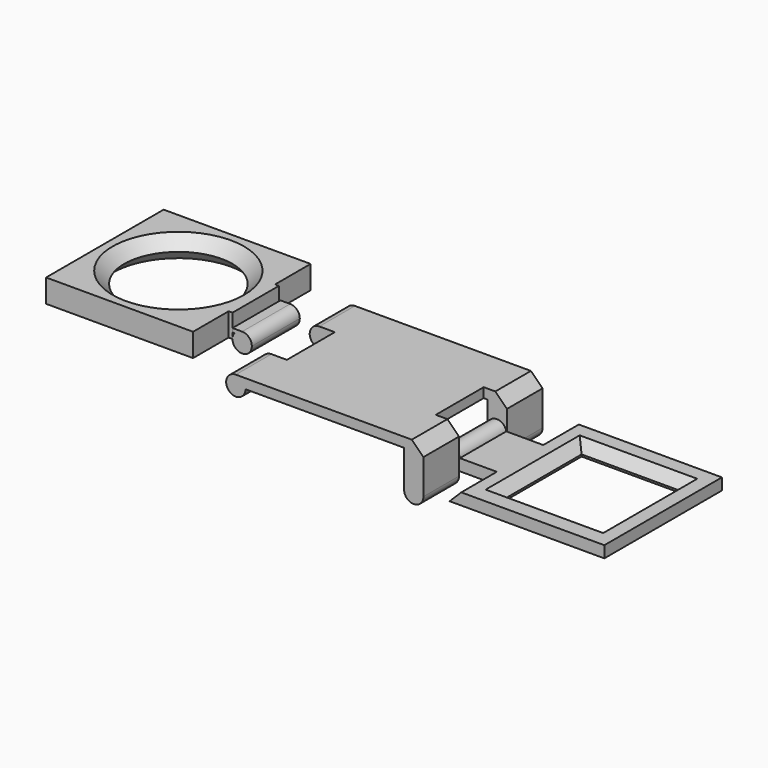
from build123d import *

# Parameters (mm, degrees)
F0_W      = 25.4
F0_H      = 25.4
F0_W_2    = 9
F0_H_2    = 15
F1_DEPTH  = 3
F2_SIZE   = 2.99999
F3_SIZE   = 2.5
F4_R      = 2.5
F5_DEPTH  = 15
F6_W      = 5
F6_H      = 11.5
F7_DEPTH  = 2.5
F8_DEPTH  = 12
F9_R      = 2.5
F10_DEPTH = 11.5
F11_R     = 2.5
F12_DEPTH = 11.5
F13_SIZE  = 3
F14_R     = 2.5
F15_DEPTH = 11.5
F16_R     = 2.5
F17_DEPTH = 11.5
F19_R     = 14
F19_W     = 1
F19_H     = 15
F20_DEPTH = 6
F22_DEPTH = 15.5
F23_SIZE  = 2.99999


# Not quite as in the source:
# - a fillet or chamfer is up to 0.001 mm smaller than in the source, because OpenCascade refuses the exact size


with BuildPart() as f1:
    # F0 (on Top) → F1 (new body)
    with BuildSketch(Plane.XY):
        Polygon((20, -19), (20, 19), (-20, 19), (-20, 7.5), (-20, -7.5), (-20, -19), align=None)
        with Locations((1.3, 0.2)):
            Rectangle(F0_W, F0_H, mode=Mode.SUBTRACT)
        with Locations((-24.5, 0)):
            Rectangle(F0_W_2, F0_H_2)
    extrude(amount=F1_DEPTH)

    # F2 (size 3 in the source; OpenCascade refuses exactly that, so slightly less here)
    f2_edges = [f1.edges().sort_by_distance(p)[0] for p in [
        (-20, -13.25, 3),
        (-20, 13.25, 3),
    ]]
    chamfer(f2_edges, length=F2_SIZE)

    # F3
    f3_edges = [f1.edges().sort_by_distance(p)[0] for p in [
        (1.3, 12.9, 3),
        (14, 0.2, 3),
        (1.3, -12.5, 3),
        (-11.4, 0.2, 3),
    ]]
    chamfer(f3_edges, length=F3_SIZE)

    # F4 (on face) → F5 (join)
    with BuildSketch(Plane.XZ.offset(7.5)):
        with Locations((-29, 2.5)):
            Circle(F4_R)
    extrude(amount=-F5_DEPTH)


with BuildPart() as f7:
    # F6 (on Top) → F7 (new body)
    with BuildSketch(Plane.XY):
        Polygon((19.25, 19.25), (-24.25, 19.25), (-24.25, 7.75), (-20.25, 7.75), (-20.25, -7.75), (-24.25, -7.75), (-24.25, -19.25), (19.25, -19.25), (19.25, -7.75), (18.25, -7.75), (18.25, 7.75), (19.25, 7.75), align=None)
        with Locations((21.75, -13.5)):
            Rectangle(F6_W, F6_H)
        with Locations((21.75, 13.5)):
            Rectangle(F6_W, F6_H)
    extrude(amount=-F7_DEPTH)

    # F6 (on Top) → F8 (join)
    with BuildSketch(Plane.XY):
        with Locations((21.75, -13.5)):
            Rectangle(F6_W, F6_H)
        with Locations((21.75, 13.5)):
            Rectangle(F6_W, F6_H)
    extrude(amount=-F8_DEPTH)

    # F9 (on face) → F10 (join)
    with BuildSketch(Plane.XZ.offset(19.25)):
        with Locations((21.75, -12)):
            Circle(F9_R)
    extrude(amount=-F10_DEPTH)

    # F11 (on face) → F12 (join)
    with BuildSketch(Plane(origin=(0, 19.25, 0), x_dir=(-1, 0, 0), z_dir=(0, 1, 0))):
        with Locations((-21.75, -12)):
            Circle(F11_R)
    extrude(amount=-F12_DEPTH)

    # F13
    f13_edges = [f7.edges().sort_by_distance(p)[0] for p in [
        (24.25, -13.5, 0),
        (24.25, 13.5, 0),
    ]]
    chamfer(f13_edges, length=F13_SIZE)

    # F14 (on face) → F15 (join)
    with BuildSketch(Plane.XZ.offset(19.25)):
        with Locations((-24.25, -2.5)):
            Circle(F14_R)
    extrude(amount=-F15_DEPTH)

    # F16 (on face) → F17 (join)
    with BuildSketch(Plane(origin=(0, 19.25, 0), x_dir=(-1, 0, 0), z_dir=(0, 1, 0))):
        with Locations((24.25, -2.5)):
            Circle(F16_R)
    extrude(amount=-F17_DEPTH)


with BuildPart() as f1_1:
    # F18: moved
    add(f1.part.moved(Location((50.83962, 0, -11))))


with BuildPart() as f20:
    # F19 (on Top) → F20 (new body)
    with BuildSketch(Plane.XY):
        Polygon((-35.5119029816, 7.5), (-35.5119029816, 19), (-73.5119029816, 19), (-73.5119029816, -19), (-35.5119029816, -19), (-35.5119029816, -7.5), (-36.5119029816, -7.5), (-36.5119029816, 7.5), align=None)
        with Locations((-54.5119029816, 0)):
            Circle(F19_R, mode=Mode.SUBTRACT)
        with Locations((-35.0119029816, 0)):
            Rectangle(F19_W, F19_H)
        with Locations((-36.0119029816, 0)):
            Rectangle(F19_W, F19_H)
    extrude(amount=F20_DEPTH)

    # F23 (size 3 in the source; OpenCascade refuses exactly that, so slightly less here)
    f23_edges = [f20.edges().sort_by_distance(p)[0] for p in [
        (-68.511903, 0, 6),
        (-68.511903, 0, 0),
    ]]
    chamfer(f23_edges, length=F23_SIZE)


with BuildPart() as f22:
    # F21 (on face) → F22 (new body)
    with BuildSketch(Plane.XZ.offset(7.5)):
        with BuildLine():
            Line((-34.5119029816, 1), (-34.5119029816, 0))
            Line((-34.5119029816, 0), (-34.0122029705, 0))
            ThreePointArc((-34.0122029705, 0), (-33.1301028007, 0.736135063), (-32.0119029816, 1))
            Line((-32.0119029816, 1), (-34.5119029816, 1))
        make_face()
        with BuildLine():
            Line((-32.0119029816, 0), (-34.0122029705, 0))
            ThreePointArc((-34.0122029705, 0), (-32.8027723614, -3.8717082307), (-29.512202957, -1.499999982))
            ThreePointArc((-29.512202957, -1.499999982), (-30.2443299499, 0.2676609104), (-32.0119029816, 1))
            Line((-32.0119029816, 1), (-32.0119029816, 0))
        make_face()
        with BuildLine():
            ThreePointArc((-32.0119029816, 1), (-33.1301028007, 0.736135063), (-34.0122029705, 0))
            Line((-34.0122029705, 0), (-32.0119029816, 0))
            Line((-32.0119029816, 0), (-32.0119029816, 1))
        make_face()
    extrude(amount=-F22_DEPTH)


with BuildPart() as f22_1:
    # F24: moved
    add(f22.part.moved(Location((0, 0, 1.5))))


solid = Compound([f7.part, f1_1.part, f20.part, f22_1.part])
